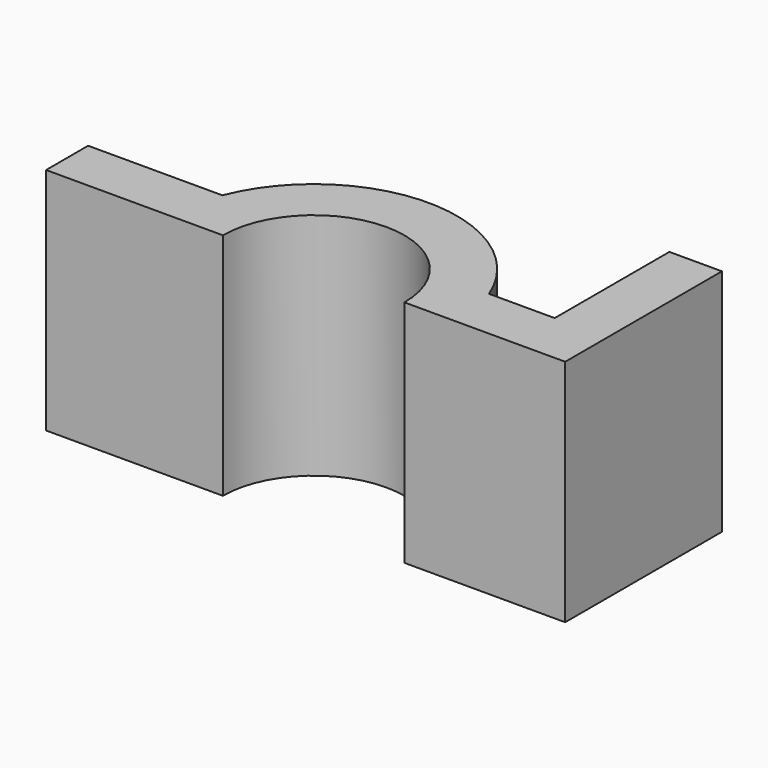
from build123d import *

# Parameters (mm, degrees)
F0_W     = 279.4
F0_H     = 279.4
F0_H_2   = 762
F1_DEPTH = 1219.2


with BuildPart() as f1:
    # F0 (on Top) → F1 (new body)
    with BuildSketch(Plane.XY):
        with BuildLine():
            Line((482.6, 0), (762, 0))
            ThreePointArc((762, 0), (748.6145632978, 142.1978748731), (708.9285154372, 279.4))
            ThreePointArc((708.9285154372, 279.4), (0, 762), (-708.9285154372, 279.4))
            Line((-708.9285154372, 279.4), (-393.4951079747, 279.4))
            ThreePointArc((-393.4951079747, 279.4), (146.6322285369, 459.7844598878), (482.6, 0))
        make_face()
        with BuildLine():
            ThreePointArc((708.9285154372, 279.4), (748.6145632978, 142.1978748731), (762, 0))
            Line((762, 0), (1057.7820539474, 0))
            Line((1057.7820539474, 0), (1057.7820539474, 279.4))
            Line((1057.7820539474, 279.4), (708.9285154372, 279.4))
        make_face()
        with Locations((1197.4820539474, 139.7)):
            Rectangle(F0_W, F0_H)
        with BuildLine():
            Line((-393.4951079747, 279.4), (-708.9285154372, 279.4))
            ThreePointArc((-708.9285154372, 279.4), (-748.6145632978, 142.1978748731), (-762, 0))
            Line((-762, 0), (-482.6, 0))
            ThreePointArc((-482.6, 0), (-459.7844598878, 146.6322285369), (-393.4951079747, 279.4))
        make_face()
        with BuildLine():
            ThreePointArc((-762, 0), (-748.6145632978, 142.1978748731), (-708.9285154372, 279.4))
            Line((-708.9285154372, 279.4), (-1422.4, 279.4))
            Line((-1422.4, 279.4), (-1422.4, 0))
            Line((-1422.4, 0), (-762, 0))
        make_face()
        with Locations((1197.4820539474, 660.4)):
            Rectangle(F0_W, F0_H_2)
    extrude(amount=F1_DEPTH)


solid = f1.part
